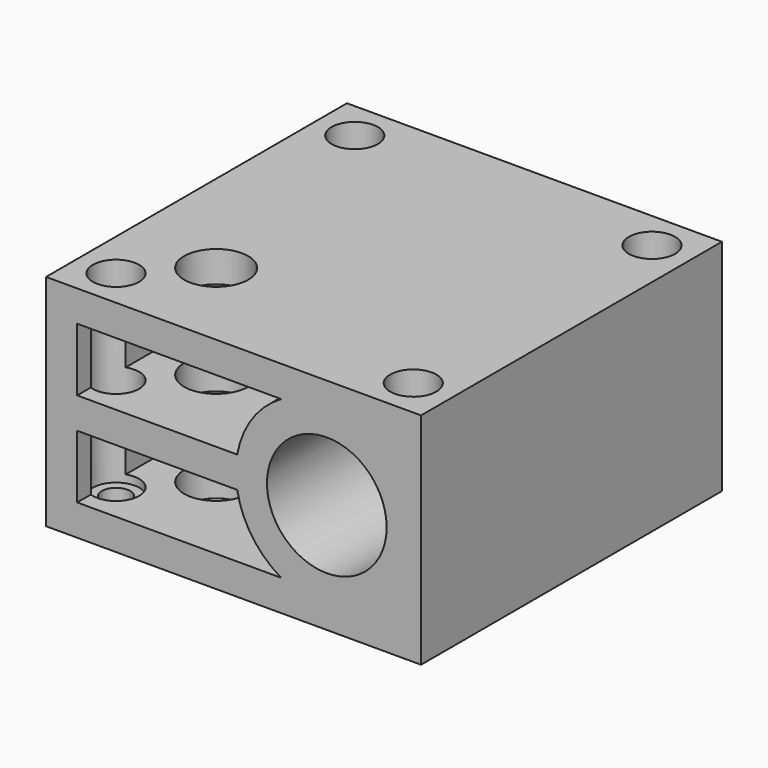
from build123d import *

# Parameters (mm, degrees)
F2_W     = 48.25
F2_H     = 28.25
F2_R     = 7.7
F3_DEPTH = 24.2
F5_R     = 2.975
F6_DEPTH = 25.25
F4_R     = 1.825
F7_DEPTH = 28.25
F4_R_2   = 4.125
F8_DEPTH = 28.25


# Not quite as in the source:
# - a feature names something its author has since deleted; it is built from what else it names


with BuildPart() as f3:
    # F2 (on Front) → F3 (new body, symmetric)
    with BuildSketch(Plane.XZ):
        Rectangle(F2_W, F2_H)
        with BuildLine():
            ThreePointArc((23.5277925033, 2), (23.6568686252, 1.0037000824), (23.7, 0))
            ThreePointArc((23.7, 0), (23.6568686252, -1.0037000824), (23.5277925033, -2))
            ThreePointArc((23.5277925033, -2), (22.3372126342, -5.4801491728), (20.125, -8.4186920005))
            Line((20.125, -8.4186920005), (20.125, -10.125))
            Line((20.125, -10.125), (17.8629663994, -10.125))
            ThreePointArc((17.8629663994, -10.125), (15.9935594213, -10.9973398215), (14, -11.5277925033))
            ThreePointArc((14, -11.5277925033), (12, -11.7), (10, -11.5277925033))
            ThreePointArc((10, -11.5277925033), (8.0064405787, -10.9973398215), (6.1370336006, -10.125))
            Line((6.1370336006, -10.125), (-20.125, -10.125))
            Line((-20.125, -10.125), (-20.125, -2))
            Line((-20.125, -2), (-20.125, 2))
            Line((-20.125, 2), (-20.125, 10.125))
            Line((-20.125, 10.125), (6.1370336006, 10.125))
            ThreePointArc((6.1370336006, 10.125), (8.0064405787, 10.9973398215), (10, 11.5277925033))
            ThreePointArc((10, 11.5277925033), (12, 11.7), (14, 11.5277925033))
            ThreePointArc((14, 11.5277925033), (15.9935594213, 10.9973398215), (17.8629663994, 10.125))
            Line((17.8629663994, 10.125), (20.125, 10.125))
            Line((20.125, 10.125), (20.125, 8.4186920005))
            ThreePointArc((20.125, 8.4186920005), (22.3372126342, 5.4801491728), (23.5277925033, 2))
        make_face(mode=Mode.SUBTRACT)
        with BuildLine():
            Line((14, 10.125), (14, 11.5277925033))
            ThreePointArc((14, 11.5277925033), (12, 11.7), (10, 11.5277925033))
            Line((10, 11.5277925033), (10, 10.125))
            Line((10, 10.125), (14, 10.125))
        make_face()
        with BuildLine():
            Line((20.125, 2), (20.125, 8.4186920005))
            ThreePointArc((20.125, 8.4186920005), (19.045826619, 9.3405742466), (17.8629663994, 10.125))
            Line((17.8629663994, 10.125), (14, 10.125))
            Line((14, 10.125), (10, 10.125))
            Line((10, 10.125), (6.1370336006, 10.125))
            ThreePointArc((6.1370336006, 10.125), (2.4024206149, 6.6915222444), (0.4722074967, 2))
            ThreePointArc((0.4722074967, 2), (0.3, 0), (0.4722074967, -2))
            ThreePointArc((0.4722074967, -2), (2.4024206149, -6.6915222444), (6.1370336006, -10.125))
            Line((6.1370336006, -10.125), (10, -10.125))
            Line((10, -10.125), (14, -10.125))
            Line((14, -10.125), (17.8629663994, -10.125))
            ThreePointArc((17.8629663994, -10.125), (19.045826619, -9.3405742466), (20.125, -8.4186920005))
            Line((20.125, -8.4186920005), (20.125, -2))
            Line((20.125, -2), (20.125, 2))
        make_face()
        with Locations((12, 0)):
            Circle(F2_R, mode=Mode.SUBTRACT)
        with BuildLine():
            ThreePointArc((10, -11.5277925033), (12, -11.7), (14, -11.5277925033))
            Line((14, -11.5277925033), (14, -10.125))
            Line((14, -10.125), (10, -10.125))
            Line((10, -10.125), (10, -11.5277925033))
        make_face()
        with BuildLine():
            ThreePointArc((0.4722074967, -2), (0.3, 0), (0.4722074967, 2))
            Line((0.4722074967, 2), (-20.125, 2))
            Line((-20.125, 2), (-20.125, -2))
            Line((-20.125, -2), (0.4722074967, -2))
        make_face()
        with BuildLine():
            ThreePointArc((23.5277925033, -2), (23.6568686252, -1.0037000824), (23.7, 0))
            ThreePointArc((23.7, 0), (23.6568686252, 1.0037000824), (23.5277925033, 2))
            Line((23.5277925033, 2), (20.125, 2))
            Line((20.125, 2), (20.125, -2))
            Line((20.125, -2), (23.5277925033, -2))
        make_face()
        with BuildLine():
            Line((20.125, 2), (23.5277925033, 2))
            ThreePointArc((23.5277925033, 2), (22.3372126342, 5.4801491728), (20.125, 8.4186920005))
            Line((20.125, 8.4186920005), (20.125, 2))
        make_face()
        with BuildLine():
            ThreePointArc((20.125, -8.4186920005), (22.3372126342, -5.4801491728), (23.5277925033, -2))
            Line((23.5277925033, -2), (20.125, -2))
            Line((20.125, -2), (20.125, -8.4186920005))
        make_face()
        with BuildLine():
            Line((14, 10.125), (17.8629663994, 10.125))
            ThreePointArc((17.8629663994, 10.125), (15.9935594213, 10.9973398215), (14, 11.5277925033))
            Line((14, 11.5277925033), (14, 10.125))
        make_face()
        with BuildLine():
            Line((10, 10.125), (10, 11.5277925033))
            ThreePointArc((10, 11.5277925033), (8.0064405787, 10.9973398215), (6.1370336006, 10.125))
            Line((6.1370336006, 10.125), (10, 10.125))
        make_face()
        with BuildLine():
            ThreePointArc((14, -11.5277925033), (15.9935594213, -10.9973398215), (17.8629663994, -10.125))
            Line((17.8629663994, -10.125), (14, -10.125))
            Line((14, -10.125), (14, -11.5277925033))
        make_face()
        with BuildLine():
            ThreePointArc((6.1370336006, -10.125), (8.0064405787, -10.9973398215), (10, -11.5277925033))
            Line((10, -11.5277925033), (10, -10.125))
            Line((10, -10.125), (6.1370336006, -10.125))
        make_face()
        with BuildLine():
            ThreePointArc((17.8629663994, 10.125), (19.045826619, 9.3405742466), (20.125, 8.4186920005))
            Line((20.125, 8.4186920005), (20.125, 10.125))
            Line((20.125, 10.125), (17.8629663994, 10.125))
        make_face()
        with BuildLine():
            Line((20.125, -10.125), (20.125, -8.4186920005))
            ThreePointArc((20.125, -8.4186920005), (19.045826619, -9.3405742466), (17.8629663994, -10.125))
            Line((17.8629663994, -10.125), (20.125, -10.125))
        make_face()
    extrude(amount=F3_DEPTH, both=True)

    # F5 (on face) → F6 (cut)
    with BuildSketch(Plane.XY.offset(14.125)):
        with Locations((-19.125, 19.2)):
            Circle(F5_R)
        with Locations((19.125, -19.2)):
            Circle(F5_R)
        with Locations((-19.125, -19.2)):
            Circle(F5_R)
        with Locations((19.125, 19.2)):
            Circle(F5_R)
    extrude(amount=-F6_DEPTH, mode=Mode.SUBTRACT)

    # F4 (on face) → F7 (cut)
    with BuildSketch(Plane(origin=(0, 0, -14.125), x_dir=(1, 0, 0), z_dir=(0, 0, -1))):
        with Locations((-19.125, 19.2)):
            Circle(F4_R)
        with Locations((19.125, 19.2)):
            Circle(F4_R)
        with Locations((19.125, -19.2)):
            Circle(F4_R)
        with Locations((-19.125, -19.2)):
            Circle(F4_R)
    extrude(amount=-F7_DEPTH, mode=Mode.SUBTRACT)

    # F4 (on face) → F8 (cut)
    with BuildSketch(Plane(origin=(0, 0, -14.125), x_dir=(1, 0, 0), z_dir=(0, 0, -1))):
        with Locations((-12, 12)):
            Circle(F4_R_2)
    extrude(amount=-F8_DEPTH, mode=Mode.SUBTRACT)


solid = f3.part
